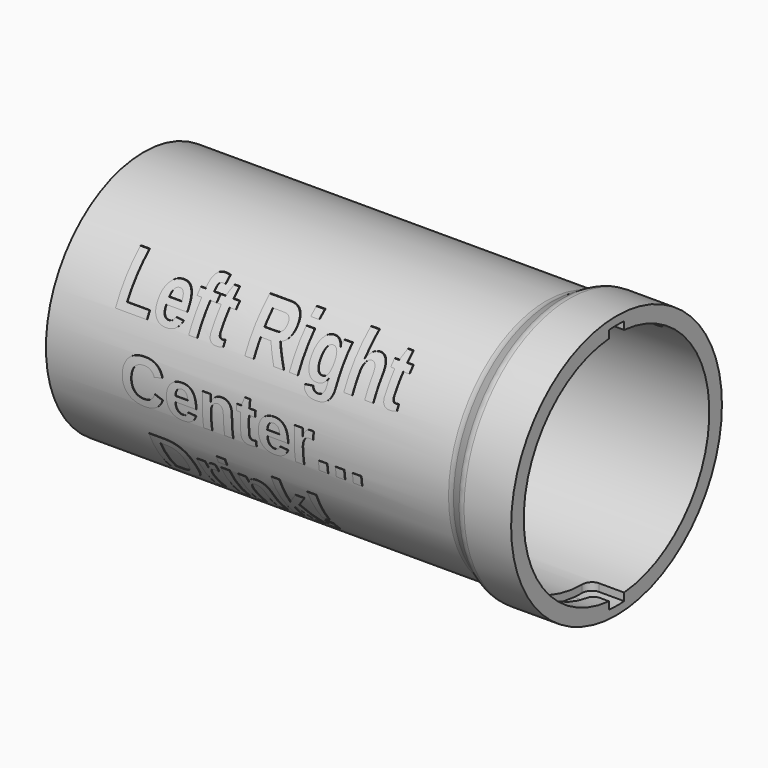
from build123d import *

# Parameters (mm, degrees)
F2_R          = 2
F4_DEPTH      = 5.5
F5_W          = 3
F5_H          = 7.349659
F6_ANGLE      = 45
F7_W          = 3
F7_H          = 8.315017
F8_ANGLE      = 45
F9_R          = 1.5
F10_R         = 1.49999
F11_R         = 1
F13_TEXT_SIZE = 9.722222
F14_DEPTH     = 20
F15_R         = 29.5
F15_R_2       = 19.5
F16_DEPTH     = 61.2
F17_DEPTH     = 74.001


# Not quite as in the source:
# - a fillet or chamfer is up to 0.001 mm smaller than in the source, because OpenCascade refuses the exact size
# - Text() gives the source's letters only with a copy of the font that has no kerning and outlines rounded to 1/6400 em; it was checked with that copy


with BuildPart() as f1:
    # F0 (on Front) → F1 (revolve)
    with BuildSketch(Plane.XZ):
        Polygon((0, 19.4), (0, 0), (1, 0), (1, 18.4), (68.5, 18.4), (75, 18.4), (75, 20.9), (67, 20.9), (64.401924, 19.4), align=None)
    revolve(axis=Axis((0.5, 0, 0), (-1, 0, 0)))

    # F2
    f2_edges = [f1.edges().sort_by_distance(p)[0] for p in [
        (67, 0, -20.9),
        (64.401924, 0, -19.4),
    ]]
    fillet(f2_edges, radius=F2_R)

    # F3 (on face) → F4 (cut)
    with BuildSketch(Plane.YZ.offset(75)):
        with BuildLine():
            Line((1.5, -19.542518), (1.5, 19.542518))
            ThreePointArc((1.5, 19.542518), (0, 19.6), (-1.5, 19.542518))
            Line((-1.5, 19.542518), (-1.5, -19.542518))
            ThreePointArc((-1.5, -19.542518), (0, -19.6), (1.5, -19.542518))
        make_face()
    extrude(amount=-F4_DEPTH, mode=Mode.SUBTRACT)

    # F5 (on Front) → F6 (revolve, cut)
    with BuildSketch(Plane.XZ):
        with Locations((71, 15.92517)):
            Rectangle(F5_W, F5_H)
    revolve(axis=Axis((71, 0, 0), (-1, 0, 0)), revolution_arc=F6_ANGLE, mode=Mode.SUBTRACT)

    # F7 (on Front) → F8 (revolve, cut)
    with BuildSketch(Plane.XZ):
        with Locations((71, -15.442491)):
            Rectangle(F7_W, F7_H)
    revolve(axis=Axis((71, 0, 0), (-1, 0, 0)), revolution_arc=F8_ANGLE, mode=Mode.SUBTRACT)

    # F9
    f9_edges = [f1.edges().sort_by_distance(p)[0] for p in [
        (69.5, -1.5, 18.940637),
        (69.5, 1.5, -18.940637),
    ]]
    fillet(f9_edges, radius=F9_R)

    # F10 (radius 1.5 in the source; OpenCascade refuses exactly that, so slightly less here)
    f10_edges = [f1.edges().sort_by_distance(p)[0] for p in [
        (69.5, 13.435029, 13.435029),
        (72.5, 13.435029, 13.435029),
        (69.5, -13.435029, -13.435029),
        (72.5, -13.435029, -13.435029),
    ]]
    fillet(f10_edges, radius=F10_R)

    # F11
    f11_edges = [f1.edges().sort_by_distance(p)[0] for p in [
        (72.5, 1.5, 18.940637),
        (72.5, -1.5, -18.940637),
    ]]
    fillet(f11_edges, radius=F11_R)

    # F13 (on Front) → F14 (join)
    with BuildSketch(Plane.XZ):
        with Locations((9.088325, 8)):
            Text('Left Right', F13_TEXT_SIZE, font='Arimo', font_style=FontStyle.BOLD, text_align=(TextAlign.LEFT, TextAlign.BOTTOM))
        with Locations((11.78928, -3.180556)):
            Text('Center...', F13_TEXT_SIZE, font='Arimo', font_style=FontStyle.BOLD, text_align=(TextAlign.LEFT, TextAlign.BOTTOM))
        with Locations((14.490234, -14.361111)):
            Text('Drink!', F13_TEXT_SIZE, font='Arimo', font_style=FontStyle.BOLD, text_align=(TextAlign.LEFT, TextAlign.BOTTOM))
    extrude(amount=F14_DEPTH)

    # F15 (on face) → F16 (cut)
    with BuildSketch(Plane(origin=(0, 0, 0), x_dir=(0, -1, 0), z_dir=(-1, 0, 0))):
        Circle(F15_R)
        Circle(F15_R_2, mode=Mode.SUBTRACT)
    extrude(amount=-F16_DEPTH, mode=Mode.SUBTRACT)

    # F17 (cut, through all): a face of the model
    f17_faces = [f1.faces().sort_by_distance(p)[0] for p in [
        (1, 0, 0),
    ]]
    extrude(f17_faces, amount=F17_DEPTH, mode=Mode.SUBTRACT)


solid = f1.part
